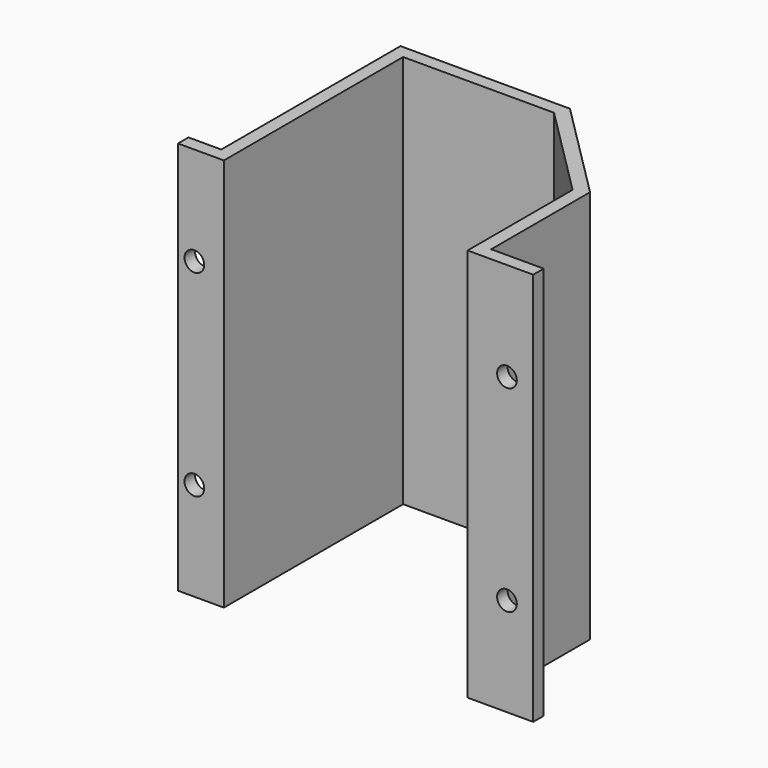
from build123d import *

# Parameters (mm, degrees)
F1_DEPTH = 60
F2_R     = 6.25
F3_DEPTH = 2
F4_DEPTH = 2
F5_R     = 1.5
F6_DEPTH = 2
F7_R     = 1.5
F8_DEPTH = 2


with BuildPart() as f1:
    # F0 (on Top) → F1 (new body)
    with BuildSketch(Plane.XY):
        Polygon((0, 2), (0, 0), (7.0000001118, 0), (7.0000001118, 34.142), (30, 34.142), (44.142, 19.9997287538), (44.142, 0), (54.142, 0), (54.142, 2), (46.142, 2), (46.142, 20.8281446432), (30.8284383602, 36.142), (5.0000001118, 36.142), (5.0000001118, 2), align=None)
    extrude(amount=F1_DEPTH)

    # F2 (on face) → F3 (cut)
    with BuildSketch(Plane(origin=(33.4855148215, 33.4848725755, 0), x_dir=(-0.7071, 0.7071135623, 0), z_dir=(0.7071135623, 0.7071, 0))):
        with Locations((-7.1303164004, 40)):
            Circle(F2_R)
    extrude(amount=-F3_DEPTH, mode=Mode.SUBTRACT)

    # F2 (on face) → F4 (cut)
    with BuildSketch(Plane(origin=(33.4855148215, 33.4848725755, 0), x_dir=(-0.7071, 0.7071135623, 0), z_dir=(0.7071135623, 0.7071, 0))):
        with Locations((-7.0707175203, 20)):
            Circle(F2_R)
    extrude(amount=-F4_DEPTH, mode=Mode.SUBTRACT)

    # F5 (on face) → F6 (cut)
    with BuildSketch(Plane(origin=(0, 2, 0), x_dir=(-1, 0, 0), z_dir=(0, 1, 0))):
        with Locations((-50.142, 45)):
            Circle(F5_R)
        with Locations((-50.142, 15)):
            Circle(F5_R)
    extrude(amount=-F6_DEPTH, mode=Mode.SUBTRACT)

    # F7 (on face) → F8 (cut)
    with BuildSketch(Plane(origin=(0, 2, 0), x_dir=(-1, 0, 0), z_dir=(0, 1, 0))):
        with Locations((-2.5000000559, 15)):
            Circle(F7_R)
        with Locations((-2.5000000559, 45)):
            Circle(F7_R)
    extrude(amount=-F8_DEPTH, mode=Mode.SUBTRACT)


solid = f1.part
